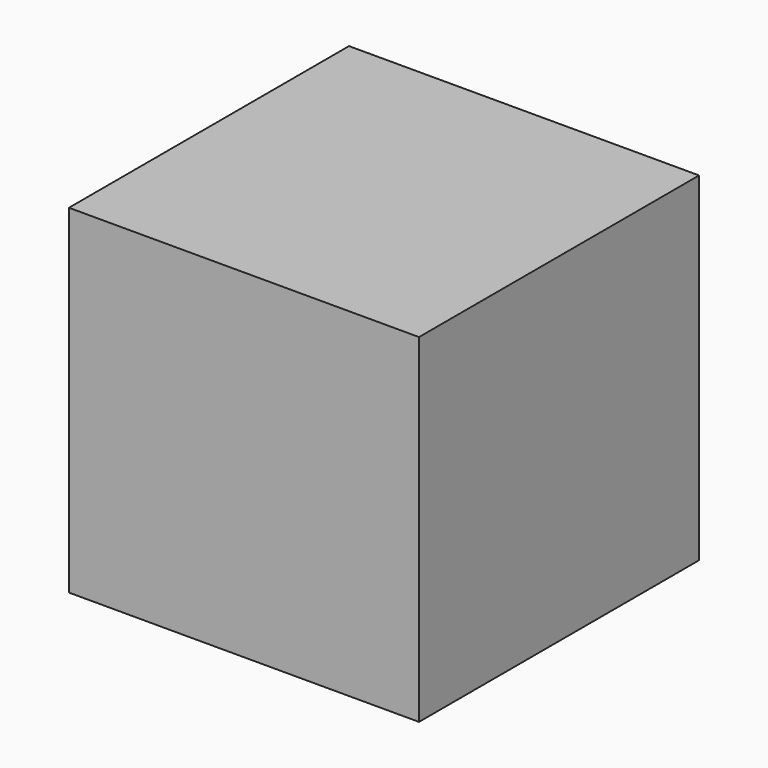
from build123d import *

# Parameters (mm, degrees)
F0_W     = 93.000068
F0_H     = 93.000068
F1_DEPTH = 90.000074


# Not quite as in the source:
# - the program builds the solid bodies; features that only make, move or delete a surface that nothing else refers to are left out


with BuildPart() as f1:
    # F0 (on Top) → F1 (new body)
    with BuildSketch(Plane.XY):
        with Locations((46.500034, 46.500034)):
            Rectangle(F0_W, F0_H)
    extrude(amount=F1_DEPTH)


solid = f1.part
